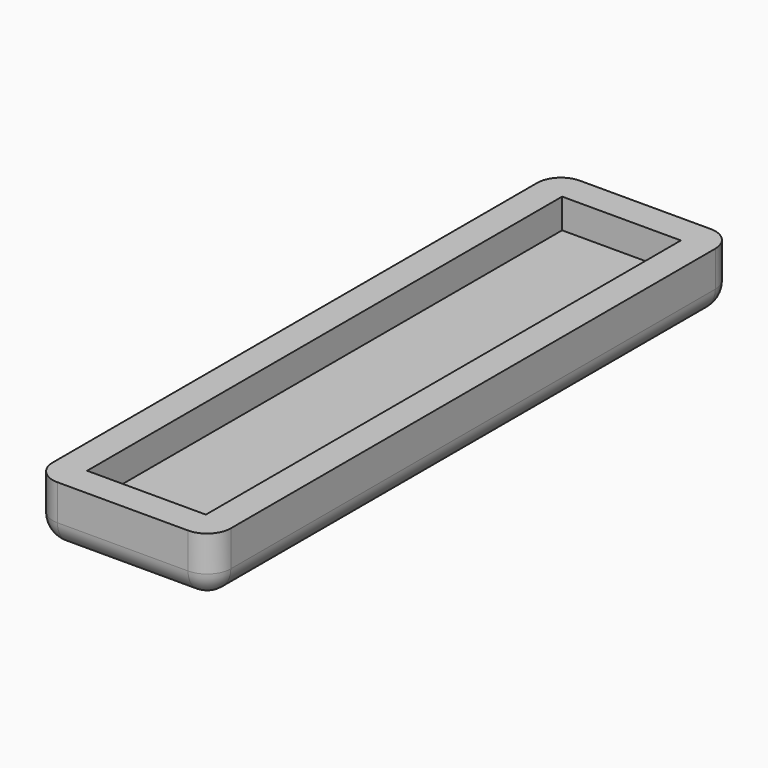
from build123d import *

# Parameters (mm, degrees)
F0_W     = 38.1
F0_H     = 139.7
F0_W_2   = 25.4
F0_H_2   = 127
F1_DEPTH = 12.7
F2_DEPTH = 6.35
F3_F1_R  = 5.08
F3_F2_R  = 5.08
F3_F3_R  = 5.08
F3_F4_R  = 5.08
F3_F5_R  = 5.08


# Not quite as in the source:
# - a feature of the source that left no trace in its solid (it failed there, or was rolled back) is left out


with BuildPart() as f1:
    # F0 (on Top) → F1 (new body)
    with BuildSketch(Plane.XY):
        Rectangle(F0_W, F0_H)
        Rectangle(F0_W_2, F0_H_2, mode=Mode.SUBTRACT)
    extrude(amount=F1_DEPTH)

    # F0 (on Top) → F2 (join)
    with BuildSketch(Plane.XY):
        Rectangle(F0_W_2, F0_H_2)
    extrude(amount=F2_DEPTH)

    # F3: fillet of radius 5.08 on 6 edges, made by hand

    # F3_f1
    f3_f1_edges = [f1.edges().sort_by_distance(p)[0] for p in [
        (19.05, -69.85, 6.35),
    ]]
    fillet(f3_f1_edges, radius=F3_F1_R)

    # F3_f2
    f3_f2_edges = [f1.edges().sort_by_distance(p)[0] for p in [
        (19.05, 69.85, 6.35),
    ]]
    fillet(f3_f2_edges, radius=F3_F2_R)

    # F3_f3
    f3_f3_edges = [f1.edges().sort_by_distance(p)[0] for p in [
        (-19.05, -69.85, 6.35),
    ]]
    fillet(f3_f3_edges, radius=F3_F3_R)

    # F3_f4
    f3_f4_edges = [f1.edges().sort_by_distance(p)[0] for p in [
        (-19.05, 69.85, 6.35),
    ]]
    fillet(f3_f4_edges, radius=F3_F4_R)

    # F3_f5
    f3_f5_edges = [f1.edges().sort_by_distance(p)[0] for p in [
        (0, 69.85, 0),
    ]]
    fillet(f3_f5_edges, radius=F3_F5_R)


solid = f1.part
